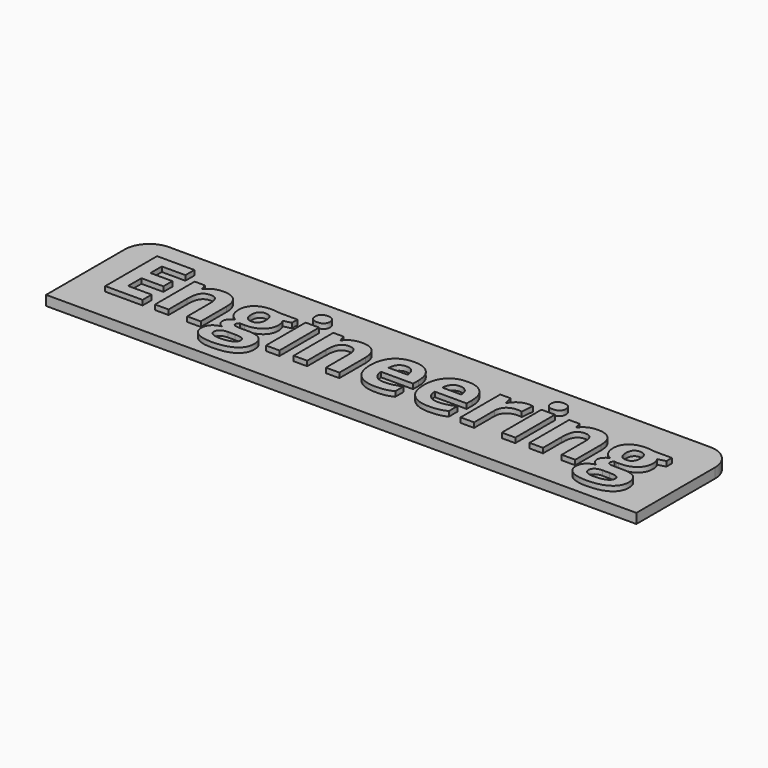
from build123d import *

# Parameters (mm, degrees)
F0_W         = 120
F0_H         = 25
F1_DEPTH     = 2
F2_TEXT_SIZE = 18.4544405998
F3_DEPTH     = 1
F4_R         = 5


# Not quite as in the source:
# - Text() gives the source's letters only with a copy of the font that has no kerning and outlines rounded to 1/6400 em; it was checked with that copy


with BuildPart() as f1:
    # F0 (on Top) → F1 (new body)
    with BuildSketch(Plane.XY):
        Rectangle(F0_W, F0_H)
    extrude(amount=F1_DEPTH)

    # F2 (on face) → F3 (join)
    with BuildSketch(Plane.XY.offset(2)):
        with Locations((-55, -5.7871972318)):
            Text('Engineering', F2_TEXT_SIZE, font='Open Sans', font_style=FontStyle.BOLD, text_align=(TextAlign.LEFT, TextAlign.BOTTOM))
    extrude(amount=F3_DEPTH)

    # F4
    f4_edges = [f1.edges().sort_by_distance(p)[0] for p in [
        (-60, 12.5, 1),
        (60, 12.5, 1),
    ]]
    fillet(f4_edges, radius=F4_R)


solid = f1.part
